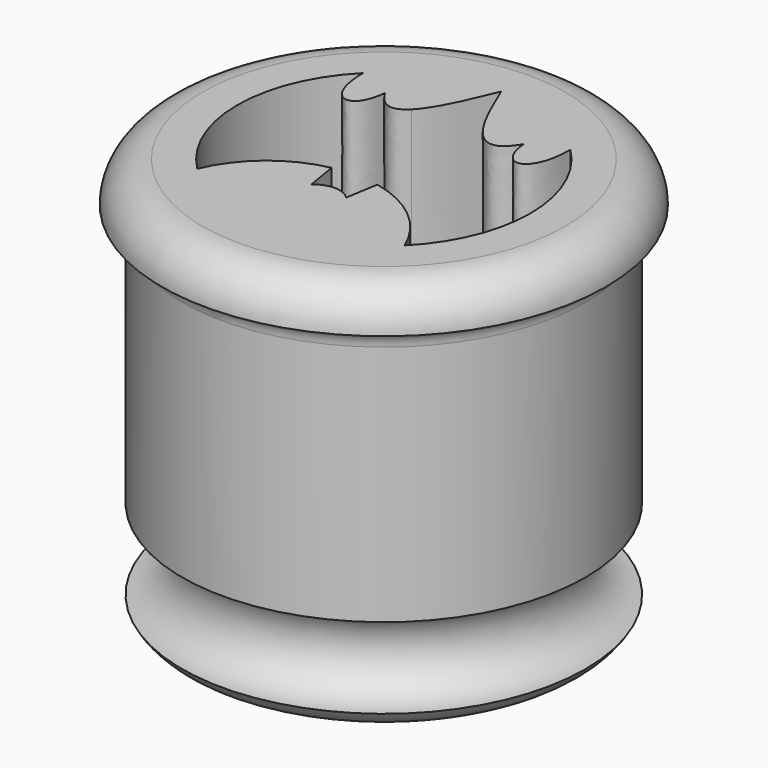
from build123d import *

# Parameters (mm, degrees)
F0_W     = 3.5
F0_H     = 10
F4_DEPTH = 25


# Not quite as in the source:
# - a fillet or chamfer that OpenCascade refuses, or shapes differently, is made with other operations: its cross-section is extruded or revolved along the edge and cut away or added


with BuildPart() as f1:
    # F0 (on Front) → F1 (revolve)
    with BuildSketch(Plane.XZ):
        with BuildLine():
            add(Edge.make_bspline(
                [(5, 10), (4.0942793712, 10), (3.5, 3.2143939752), (3.5, 0)],
                knots=[0, 0, 0, 0, 10.1118742081, 10.1118742081, 10.1118742081, 10.1118742081], degree=3))
            Line((3.5, 0), (5, 0))
            Line((5, 0), (5, 0.5))
            ThreePointArc((5, 0.5), (4, 1.5), (5, 2.5))
            Line((5, 2.5), (5, 8.5))
            ThreePointArc((5, 8.5), (5.1464466094, 8.8535533906), (5.5, 9))
            Line((5.5, 9), (5.5, 10))
            Line((5.5, 10), (5, 10))
        make_face()
        with Locations((1.75, 5)):
            Rectangle(F0_W, F0_H)
        with BuildLine():
            Line((3.5, 10), (3.5, 0))
            add(Edge.make_bspline(
                [(5, 10), (4.0942793712, 10), (3.5, 3.2143939752), (3.5, 0)],
                knots=[0, 0, 0, 0, 10.1118742081, 10.1118742081, 10.1118742081, 10.1118742081], degree=3))
            Line((5, 10), (3.5, 10))
        make_face()
    revolve(axis=Axis((0, 0, 5), (0, 0, 1)))

    # F2: fillet of radius 1 on 2 edges, made by hand

    # F2_s1 → F2_t2 (revolve, cut)
    with BuildSketch(Plane.XZ):
        with BuildLine():
            ThreePointArc((5, 0.5), (4.6339745962, 0.1339745962), (4.1339745962, 0))
            Line((4.1339745962, 0), (5, 0))
            Line((5, 0), (5, 0.5))
        make_face()
    revolve(axis=Axis((0, 0, 0), (0, 0, 1)), mode=Mode.SUBTRACT)

    # F2_s3 → F2_t4 (revolve, cut)
    with BuildSketch(Plane.XZ):
        with BuildLine():
            ThreePointArc((5.5, 9), (5.2071067812, 9.7071067812), (4.5, 10))
            Line((4.5, 10), (5.5, 10))
            Line((5.5, 10), (5.5, 9))
        make_face()
    revolve(axis=Axis((0, 0, 10), (0, 0, 1)), mode=Mode.SUBTRACT)

    # F3 (on face) → F4 (cut)
    with BuildSketch(Plane(origin=(0, 0, 0), x_dir=(1, 0, 0), z_dir=(0, 0, -1))):
        with BuildLine():
            ThreePointArc((2.5696080796, -2.5696080796), (3.3573547511, -1.3906618716), (3.6339745962, 0))
            ThreePointArc((3.6339745962, 0), (3.3573547511, 1.3906618716), (2.5696080796, 2.5696080796))
            ThreePointArc((2.5696080796, 2.5696080796), (1.7735963788, 1.4915186107), (0.5658317976, 0.9108153755))
            ThreePointArc((0.5658317976, 0.9108153755), (0.2844067223, 0.8672301951), (0, 0.852650853))
            ThreePointArc((0, 0.852650853), (-0.2844067223, 0.8672301951), (-0.5658317976, 0.9108153755))
            ThreePointArc((-0.5658317976, 0.9108153755), (-1.7735963788, 1.4915186107), (-2.5696080796, 2.5696080796))
            ThreePointArc((-2.5696080796, 2.5696080796), (-3.6339745962, 0), (-2.5696080796, -2.5696080796))
            add(Edge.make_bspline(
                [(-2.5696080796, -2.5696080796), (-2.5696080796, -1.2858674651), (-1.8195327018, -1.1542756278), (-1.7160946607, -2.1836098922)],
                knots=[0, 0, 0, 0, 0.9367388948, 0.9367388948, 0.9367388948, 0.9367388948], degree=3))
            add(Edge.make_bspline(
                [(-1.7160946607, -2.1836098922), (-1.4292562782, -1.6936314013), (-1.1484208124, -1.7084361716), (-0.8862952606, -1.9693091494)],
                knots=[0, 0, 0, 0, 0.986714465, 0.986714465, 0.986714465, 0.986714465], degree=3))
            ThreePointArc((-0.8862952606, -1.9693091494), (0, -1.8935369514), (0.8862952606, -1.9693091494))
            add(Edge.make_bspline(
                [(1.7160946607, -2.1836098922), (1.4292562782, -1.6936314013), (1.1484208124, -1.7084361716), (0.8862952606, -1.9693091494)],
                knots=[0, 0, 0, 0, 0.986714465, 0.986714465, 0.986714465, 0.986714465], degree=3))
            add(Edge.make_bspline(
                [(2.5696080796, -2.5696080796), (2.5696080796, -1.2858674651), (1.8195327018, -1.1542756278), (1.7160946607, -2.1836098922)],
                knots=[0, 0, 0, 0, 0.9367388948, 0.9367388948, 0.9367388948, 0.9367388948], degree=3))
        make_face()
        with BuildLine():
            ThreePointArc((0, 0.852650853), (0.2844067223, 0.8672301951), (0.5658317976, 0.9108153755))
            Line((0.5658317976, 0.9108153755), (0.4351094112, 1.7111294663))
            ThreePointArc((0.4351094112, 1.7111294663), (0, 1.5309012471), (-0.4351094112, 1.7111294663))
            Line((-0.4351094112, 1.7111294663), (-0.5658317976, 0.9108153755))
            ThreePointArc((-0.5658317976, 0.9108153755), (-0.2844067223, 0.8672301951), (0, 0.852650853))
        make_face()
        with BuildLine():
            add(Edge.make_bspline(
                [(-0.8862952606, -1.9693091494), (-0.5515220121, -2.3024826748), (-0.2472666579, -3.0370200771), (0, -3.6339745962)],
                knots=[0.986714465, 0.986714465, 0.986714465, 0.986714465, 2.2468953379, 2.2468953379, 2.2468953379, 2.2468953379], degree=3))
            add(Edge.make_bspline(
                [(0.8862952606, -1.9693091494), (0.5515220121, -2.3024826748), (0.2472666579, -3.0370200771), (0, -3.6339745962)],
                knots=[0.986714465, 0.986714465, 0.986714465, 0.986714465, 2.2468953379, 2.2468953379, 2.2468953379, 2.2468953379], degree=3))
            ThreePointArc((0.8862952606, -1.9693091494), (0, -1.8935369514), (-0.8862952606, -1.9693091494))
        make_face()
    extrude(amount=-F4_DEPTH, mode=Mode.SUBTRACT)


solid = f1.part
